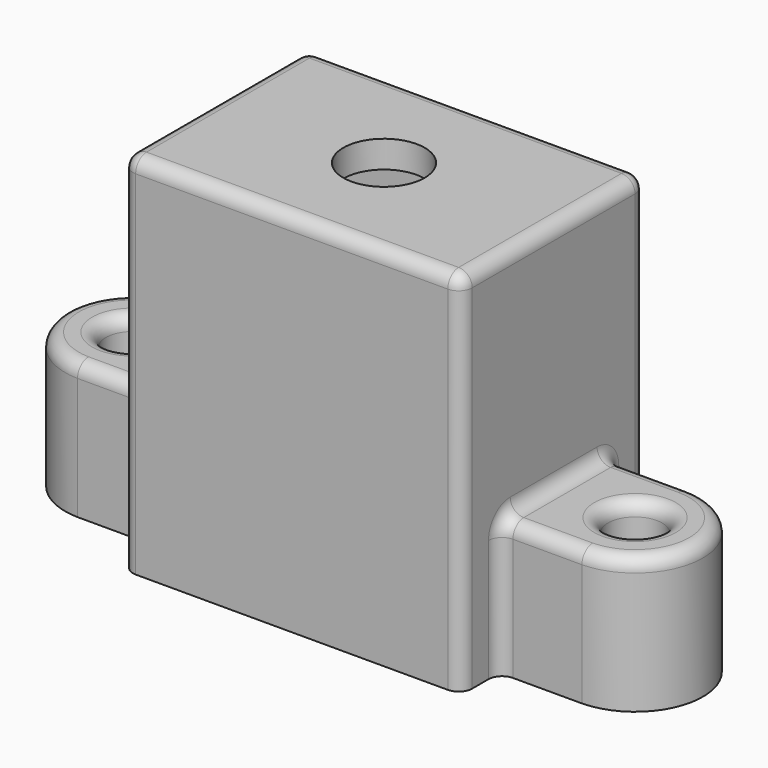
from build123d import *

# Parameters (mm, degrees)
F0_W     = 25
F0_H     = 17
F1_DEPTH = 27
F2_W     = 21
F2_H     = 13
F3_DEPTH = 25
F4_R     = 2
F5_DEPTH = 10
F6_R     = 3
F7_DEPTH = 27.001
F8_R     = 1


with BuildPart() as f1:
    # F0 (on Top) → F1 (new body)
    with BuildSketch(Plane.XY):
        Rectangle(F0_W, F0_H)
    extrude(amount=F1_DEPTH)

    # F2 (on face) → F3 (cut)
    with BuildSketch(Plane(origin=(0, 0, 0), x_dir=(1, 0, 0), z_dir=(0, 0, -1))):
        Rectangle(F2_W, F2_H)
    extrude(amount=-F3_DEPTH, mode=Mode.SUBTRACT)

    # F4 (on Top) → F5 (join)
    with BuildSketch(Plane.XY):
        with BuildLine():
            Line((12.5, -4.9992689166), (18.4144997112, -4.9992689166))
            Line((18.4144997112, -4.9992689166), (18.5855002888, -4.9992689166))
            ThreePointArc((18.5855002888, -4.9992689166), (23.4998172258, 0.0427517072), (18.5, 5))
            Line((18.5, 5), (12.5, 5))
            Line((12.5, 5), (12.5, -4.9992689166))
        make_face()
        with Locations((18.5, 0)):
            Circle(F4_R, mode=Mode.SUBTRACT)
        with BuildLine():
            Line((-18.5855002888, -4.9992689166), (-18.4144997112, -4.9992689166))
            Line((-18.4144997112, -4.9992689166), (-12.5, -4.9992689166))
            Line((-12.5, -4.9992689166), (-12.5, 5))
            Line((-12.5, 5), (-18.5, 5))
            ThreePointArc((-18.5, 5), (-23.4998172258, 0.0427517072), (-18.5855002888, -4.9992689166))
        make_face()
        with Locations((-18.5, 0)):
            Circle(F4_R, mode=Mode.SUBTRACT)
    extrude(amount=F5_DEPTH)

    # F6 (on face) → F7 (cut, through all)
    with BuildSketch(Plane.XY.offset(27)):
        Circle(F6_R)
    extrude(amount=-F7_DEPTH, mode=Mode.SUBTRACT)

    # F8
    f8_edges = [f1.edges().sort_by_distance(p)[0] for p in [
        (12.5, 8.5, 13.5),
        (-12.5, 8.5, 13.5),
        (12.5, -8.5, 13.5),
        (-12.5, -8.5, 13.5),
        (-12.5, 0, 27),
        (0, -8.5, 27),
        (12.5, 0, 27),
        (0, 8.5, 27),
        (15.5, 5, 10),
        (12.5, 0.000366, 10),
        (15.54275, -4.999269, 10),
        (23.499817, 0.042752, 10),
        (16.5, 0, 10),
        (-23.499817, 0.042752, 10),
        (-15.54275, -4.999269, 10),
        (-12.5, 0.000366, 10),
        (-15.5, 5, 10),
        (-20.5, 0, 10),
        (-12.5, 5, 5),
        (-12.5, -4.999269, 5),
        (12.5, -4.999269, 5),
        (12.5, 5, 5),
    ]]
    fillet(f8_edges, radius=F8_R)


solid = f1.part
